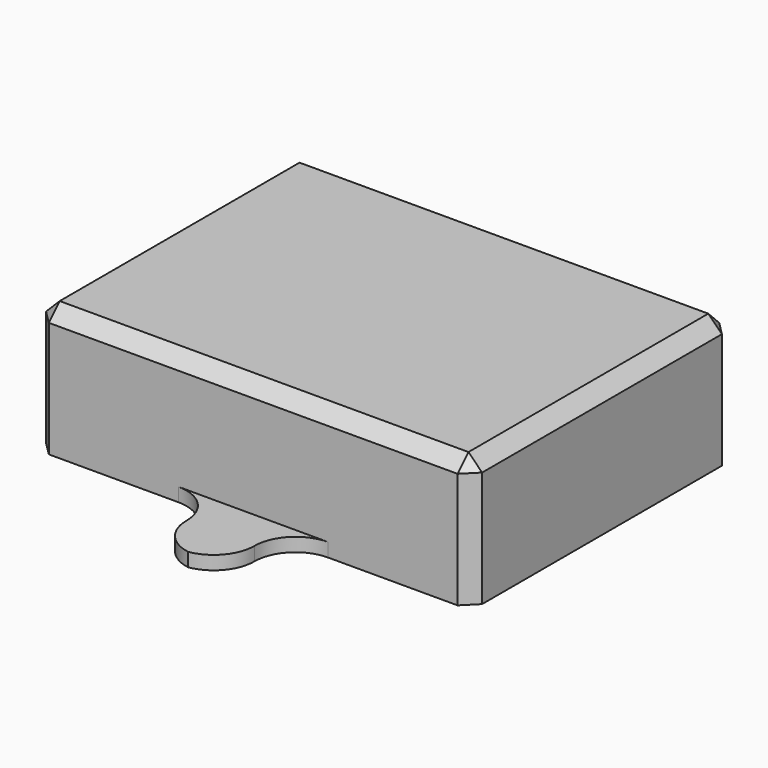
from build123d import *

# Parameters (mm, degrees)
F0_W        = 5
F0_H        = 6
F1_DEPTH    = 9.5
F2_DEPTH    = 1
F3_T1_DEPTH = 1
F3_T3_DEPTH = 16
F4_SIZE     = 1


# Not quite as in the source:
# - a fillet or chamfer that OpenCascade refuses, or shapes differently, is made with other operations: its cross-section is extruded or revolved along the edge and cut away or added


with BuildPart() as f1:
    # F0 (on Top) → F1 (new body)
    with BuildSketch(Plane.XY):
        Polygon((16, -12), (16, 12), (2.5, 12), (2.5, 6), (-2.5, 6), (-2.5, 12), (-16, 12), (-16, -12), (-2.5, -12), (-2.5, -6), (2.5, -6), (2.5, -12), align=None)
        with Locations((0, -9)):
            Rectangle(F0_W, F0_H)
        with Locations((0, 9)):
            Rectangle(F0_W, F0_H)
    extrude(amount=F1_DEPTH)

    # F0 (on Top) → F2 (join)
    with BuildSketch(Plane.XY):
        with Locations((0, 15)):
            Rectangle(F0_W, F0_H)
        with Locations((0, -15)):
            Rectangle(F0_W, F0_H)
    extrude(amount=F2_DEPTH)

    # F3: fillet of radius 3 on 8 edges, made by hand

    # F3_s2 → F3_t1 (join)
    with BuildSketch(Plane.XY):
        with BuildLine():
            ThreePointArc((5.5, -12), (3.3786796564, -12.8786796564), (2.5, -15))
            Line((2.5, -15), (2.5, -12))
            Line((2.5, -12), (5.5, -12))
        make_face()
        with BuildLine():
            ThreePointArc((-5.5, -12), (-3.3786796564, -12.8786796564), (-2.5, -15))
            Line((-2.5, -15), (-2.5, -12))
            Line((-2.5, -12), (-5.5, -12))
        make_face()
        with BuildLine():
            ThreePointArc((-5.5, 12), (-3.3786796564, 12.8786796564), (-2.5, 15))
            Line((-2.5, 15), (-2.5, 12))
            Line((-2.5, 12), (-5.5, 12))
        make_face()
        with BuildLine():
            ThreePointArc((5.5, 12), (3.3786796564, 12.8786796564), (2.5, 15))
            Line((2.5, 15), (2.5, 12))
            Line((2.5, 12), (5.5, 12))
        make_face()
    extrude(amount=F3_T1_DEPTH)

    # F3_s4 → F3_t3 (cut)
    with BuildSketch(Plane.XY.offset(-7.5)):
        with BuildLine():
            ThreePointArc((0.5, -18), (-1.6213203436, -17.1213203436), (-2.5, -15))
            Line((-2.5, -15), (-2.5, -18))
            Line((-2.5, -18), (0.5, -18))
        make_face()
        with BuildLine():
            ThreePointArc((2.5, -15), (1.6213203436, -17.1213203436), (-0.5, -18))
            Line((-0.5, -18), (2.5, -18))
            Line((2.5, -18), (2.5, -15))
        make_face()
        with BuildLine():
            ThreePointArc((-2.5, 15), (-1.6213203436, 17.1213203436), (0.5, 18))
            Line((0.5, 18), (-2.5, 18))
            Line((-2.5, 18), (-2.5, 15))
        make_face()
        with BuildLine():
            ThreePointArc((-0.5, 18), (1.6213203436, 17.1213203436), (2.5, 15))
            Line((2.5, 15), (2.5, 18))
            Line((2.5, 18), (-0.5, 18))
        make_face()
    extrude(amount=F3_T3_DEPTH, mode=Mode.SUBTRACT)

    # F4
    f4_edges = [f1.edges().sort_by_distance(p)[0] for p in [
        (-16, 0, 9.5),
        (0, 12, 9.5),
        (0, -12, 9.5),
        (16, 0, 9.5),
        (-16, 12, 4.75),
        (-16, -12, 4.75),
        (16, -12, 4.75),
        (16, 12, 4.75),
    ]]
    chamfer(f4_edges, length=F4_SIZE)


solid = f1.part
